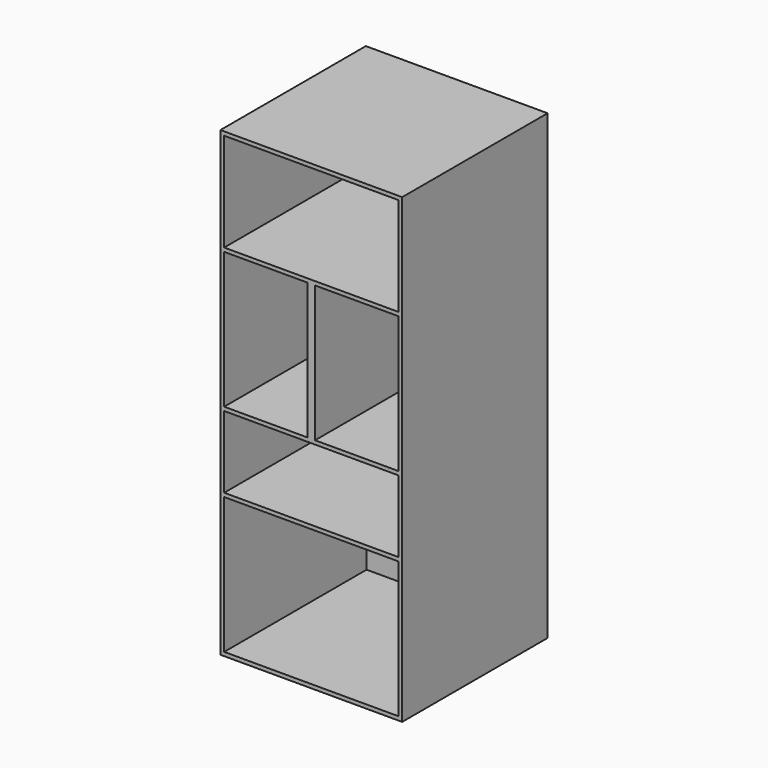
from build123d import *

# Parameters (mm, degrees)
F0_W      = 609.6
F0_H      = 609.6
F1_DEPTH  = 482.6
F2_T      = -12.7
F3_DEPTH  = 254
F4_T      = -12.7
F5_W      = 304.8
F5_H      = 609.6
F6_DEPTH  = 469.9
F7_T      = -12.7
F8_DEPTH  = 469.9
F9_DEPTH  = 342.9
F10_W     = 279.4
F10_H     = 457.2
F11_DEPTH = 596.9
F12_W     = 584.2
F12_H     = 330.2
F13_DEPTH = 596.9
F14_W     = 609.6
F14_H     = 1549.4
F15_DEPTH = 12.7


# Not quite as in the source:
# - a shell that OpenCascade refuses in one call is made with other operations: the cavity is built on its own and cut out


with BuildPart() as f1:
    # F0 (on Top) → F1 (new body)
    with BuildSketch(Plane.XY):
        with Locations((3.9980113506, 30.8666436833)):
            Rectangle(F0_W, F0_H)
    extrude(amount=F1_DEPTH)

    # F2
    f2_openings = [f1.faces().sort_by_distance(p)[0] for p in [
        (3.998011, -273.933356, 241.3),
    ]]
    offset(amount=F2_T, openings=f2_openings)

    # F3 (add): a face of the model
    f3_faces = [f1.faces().sort_by_distance(p)[0] for p in [
        (3.9980113506, 30.8666436833, 482.6),
    ]]
    extrude(f3_faces, amount=F3_DEPTH)

    # F4: a shell. OpenCascade refuses it in one call, so the cavity is built on its own and cut out:
    # the body offset inwards by the wall thickness, plus a prism from it out through each open face.
    f4_core = offset(f1.part, amount=F4_T, kind=Kind.INTERSECTION, mode=Mode.PRIVATE)
    f4_exits = [f4_core.faces().sort_by_distance(p)[0] for p in [
        (3.998011, -261.233356, 603.25),
    ]]
    add(f4_core, mode=Mode.SUBTRACT)
    extrude(f4_exits, amount=-F4_T, mode=Mode.SUBTRACT)

    # F5 (on face) → F6 (join)
    with BuildSketch(Plane.XY.offset(736.6)):
        with Locations((-148.4019886494, 30.8666436833)):
            Rectangle(F5_W, F5_H)
    extrude(amount=F6_DEPTH)

    # F7: a shell. OpenCascade refuses it in one call, so the cavity is built on its own and cut out:
    # the body offset inwards by the wall thickness, plus a prism from it out through each open face.
    f7_core = offset(f1.part, amount=F7_T, kind=Kind.INTERSECTION, mode=Mode.PRIVATE)
    f7_exits = [f7_core.faces().sort_by_distance(p)[0] for p in [
        (-148.401989, -261.233356, 965.2),
    ]]
    add(f7_core, mode=Mode.SUBTRACT)
    extrude(f7_exits, amount=-F7_T, mode=Mode.SUBTRACT)

    # F8 (add): a face of the model
    f8_faces = [f1.faces().sort_by_distance(p)[0] for p in [
        (156.3980113506, 30.8666436833, 736.6),
    ]]
    extrude(f8_faces, amount=F8_DEPTH)

    # F9 (add): a face of the model
    f9_faces = [f1.faces().sort_by_distance(p)[0] for p in [
        (3.9980113506, 30.8666436833, 1206.5),
    ]]
    extrude(f9_faces, amount=F9_DEPTH)

    # F10 (on face) → F11 (cut)
    with BuildSketch(Plane.XZ.offset(273.9333563167)):
        with Locations((156.3980113506, 965.2)):
            Rectangle(F10_W, F10_H)
    extrude(amount=-F11_DEPTH, mode=Mode.SUBTRACT)

    # F12 (on face) → F13 (cut)
    with BuildSketch(Plane.XZ.offset(273.9333563167)):
        with Locations((3.9980113506, 1371.6)):
            Rectangle(F12_W, F12_H)
    extrude(amount=-F13_DEPTH, mode=Mode.SUBTRACT)


with BuildPart() as f15:
    # F14 (on face) → F15 (new body)
    with BuildSketch(Plane.XZ.offset(273.9333563167)):
        with Locations((3.9980113506, 774.7)):
            Rectangle(F14_W, F14_H)
    extrude(amount=F15_DEPTH)


solid = f1.part
